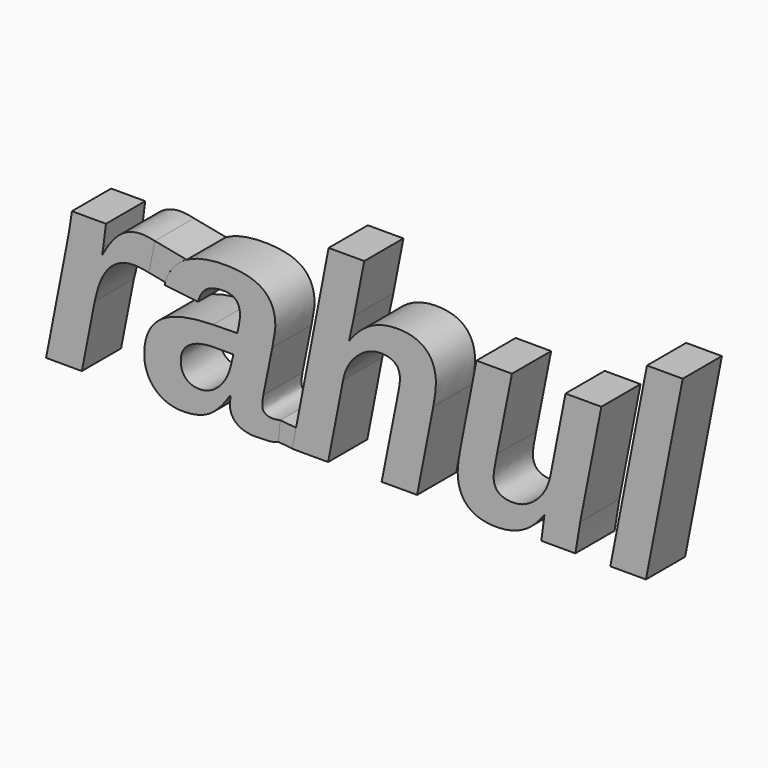
from build123d import *

# Parameters (mm, degrees)
F0_TEXT_SIZE = 150.5185185185
F1_DEPTH     = 28.33596
F1_FACE_W    = 28.33596
F1_FACE_H    = 17.5871506642
F1_FACE1_W   = 28.33596
F1_FACE1_H   = 11.4299032156


# Not quite as in the source:
# - Text() gives the source's letters only with a copy of the font that has no kerning and outlines rounded to 1/6400 em; it was checked with that copy


with BuildPart() as f1:
    # F0 (on Front) → F1 (new body)
    with BuildSketch(Plane.XZ):
        with Locations((-243.6084431065, 0)):
            Text('rahul', F0_TEXT_SIZE, font='Arimo', font_style=FontStyle.BOLDITALIC, text_align=(TextAlign.LEFT, TextAlign.BOTTOM))
    extrude(amount=F1_DEPTH)


with BuildPart() as f2:
    # F1_face (on face) → F2 (new body, up to the next surface of F1)
    with BuildSketch(Plane(origin=(-179.8850171806, -14.16798, 71.3316666667), x_dir=(0, 1, 0), z_dir=(0.9815457275, 0, -0.1912275736))):
        Rectangle(F1_FACE_W, F1_FACE_H)
    extrude(until=Until.NEXT, target=f1.part)


with BuildPart() as f3:
    # F1_face1 (on face) → F3 (new body, up to the next surface of F1)
    with BuildSketch(Plane(origin=(-106.2367764398, -14.16798, 6.5851851852), x_dir=(0, 1, 0), z_dir=(0.9958932065, 0, -0.090535746))):
        Rectangle(F1_FACE1_W, F1_FACE1_H)
    extrude(until=Until.NEXT, target=f1.part)


solid = Compound([f1.part, f2.part, f3.part])
